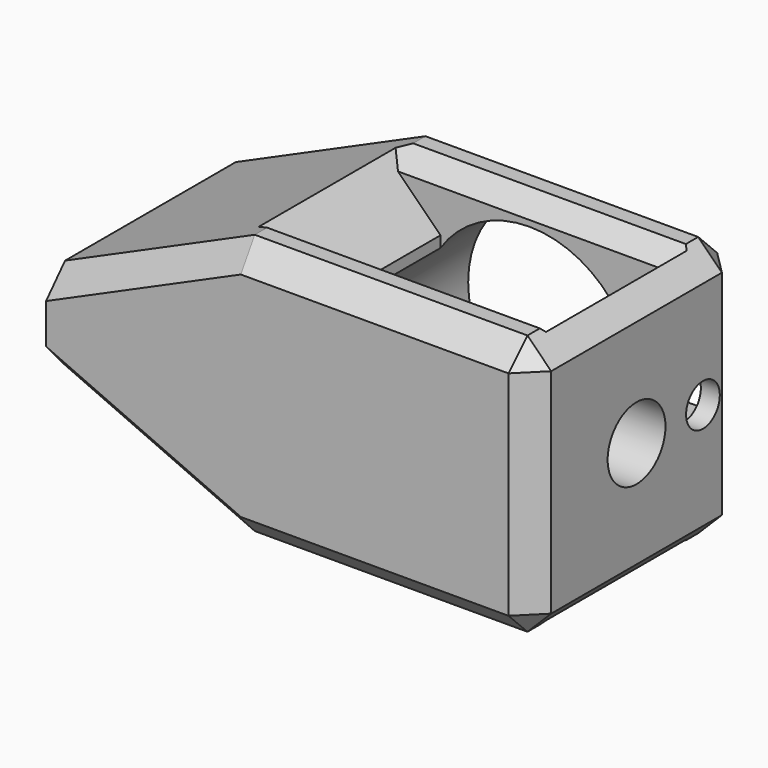
from build123d import *

# Parameters (mm, degrees)
F0_W          = 26
F0_H          = 22
F1_DEPTH      = 22
F2_R          = 9
F3_DEPTH      = 20
F4_W          = 15
F4_H          = 12.4
F5_DEPTH      = 22.001
F6_W          = 22
F6_H          = 22
F7_DEPTH      = 14
F8_W          = 18.7
F8_H          = 6
F9_DEPTH      = 12
F10_R         = 1.778
F11_DEPTH     = 40.001
F12_SIZE      = 1.5
F13_SIZE2     = 7.1236589649
F13_SIZE      = 16
F13_2_SIZE2   = 7.1236589649
F13_2_SIZE    = 16
F14_T1_DEPTH  = 27.800912408
F14_T3_DEPTH  = 27.800912408
F15_W         = 2.8
F15_H         = 5.8
F16_DEPTH     = 7
F17_W         = 22
F17_H         = 22
F18_DEPTH     = 1
F19_R         = 3.048
F20_DEPTH     = 26.5
F21_R         = 1.778
F22_DEPTH     = 6
F23_T1_DEPTH  = 2.5403411844
F23_T3_DEPTH  = 2.5403411844
F23_T5_DEPTH  = 2.5403411844
F23_T7_DEPTH  = 2.5403411844
F23_T9_DEPTH  = 32.2867319519
F23_T11_DEPTH = 32.2867319519
F23_T13_DEPTH = 30.3695452806
F24_T4_DEPTH  = 41.5282991577
F24_T10_DEPTH = 41.5282991577
F24_T16_DEPTH = 41.5282991577
F24_T22_DEPTH = 41.5282991577
F24_T28_DEPTH = 41.5282991577
F24_T34_DEPTH = 41.5282991577
F24_T40_DEPTH = 41.5282991577
F24_T46_DEPTH = 41.5282991577


# Not quite as in the source:
# - a fillet or chamfer that OpenCascade refuses, or shapes differently, is made with other operations: its cross-section is extruded or revolved along the edge and cut away or added


with BuildPart() as f1:
    # F0 (on Top) → F1 (new body)
    with BuildSketch(Plane.XY):
        with Locations((-0.9824799188, -2.7680952549)):
            Rectangle(F0_W, F0_H)
    extrude(amount=F1_DEPTH)

    # F2 (on face) → F3 (cut)
    with BuildSketch(Plane(origin=(0, 8.2319047451, 0), x_dir=(-1, 0, 0), z_dir=(0, 1, 0))):
        with Locations((0.9824799188, 11)):
            Circle(F2_R)
    extrude(amount=-F3_DEPTH, mode=Mode.SUBTRACT)

    # F4 (on face) → F5 (cut, through all)
    with BuildSketch(Plane.XY.offset(22)):
        with Locations((-0.9824799188, -2.7680952549)):
            Rectangle(F4_W, F4_H)
    extrude(amount=-F5_DEPTH, mode=Mode.SUBTRACT)

    # F6 (on face) → F7 (join)
    with BuildSketch(Plane(origin=(-13.9824799188, 0, 0), x_dir=(0, -1, 0), z_dir=(-1, 0, 0))):
        with Locations((2.7680952549, 11)):
            Rectangle(F6_W, F6_H)
    extrude(amount=F7_DEPTH)

    # F8 (on face) → F9 (cut)
    with BuildSketch(Plane(origin=(-27.9824799188, 0, 0), x_dir=(0, -1, 0), z_dir=(-1, 0, 0))):
        with Locations((2.7180952549, 11)):
            Rectangle(F8_W, F8_H)
    extrude(amount=-F9_DEPTH, mode=Mode.SUBTRACT)

    # F10 (on face) → F11 (cut, through all)
    with BuildSketch(Plane.YZ.offset(12.0175200812)):
        with Locations((-2.7180952549, 11)):
            Circle(F10_R)
    extrude(amount=-F11_DEPTH, mode=Mode.SUBTRACT)

    # F12
    f12_edges = [f1.edges().sort_by_distance(p)[0] for p in [
        (-0.98248, 3.431905, 22),
        (-0.98248, -8.968095, 22),
        (-0.98248, 3.431905, 0),
        (-0.98248, -8.968095, 0),
    ]]
    chamfer(f12_edges, length=F12_SIZE)

    # F13
    f13_edges = [f1.edges().sort_by_distance(p)[0] for p in [
        (-27.98248, -2.768095, 22),
    ]]
    f13_side = f1.faces().sort_by_distance((-10.474005, -2.768095, 22))[0]
    chamfer(f13_edges, length=F13_SIZE, length2=F13_SIZE2, reference=f13_side)

    # F13#2
    f13_2_edges = [f1.edges().sort_by_distance(p)[0] for p in [
        (-27.98248, -2.768095, 0),
    ]]
    f13_2_side = f1.faces().sort_by_distance((-10.474005, -2.768095, 0))[0]
    chamfer(f13_2_edges, length=F13_2_SIZE, length2=F13_2_SIZE2, reference=f13_2_side)

    # F14: chamfer of 2 on 4 edges, made by hand

    # F14_s2 → F14_t1 (cut)
    with BuildSketch(Plane(origin=(2.8731297183, 0, 1.2791997672), x_dir=(0, 1, 0), z_dir=(-0.9135454576, 0, -0.4067366431))):
        Polygon((8.2319047451, -22.971713726), (6.2319047451, -24.971713726), (8.2319047451, -24.971713726), align=None)
        Polygon((-11.7680952549, -24.971713726), (-13.7680952549, -22.971713726), (-13.7680952549, -24.971713726), align=None)
    extrude(amount=F14_T1_DEPTH, mode=Mode.SUBTRACT)

    # F14_s4 → F14_t3 (cut)
    with BuildSketch(Plane(origin=(-5.301463362, 0, 2.3603635629), x_dir=(0, 1, 0), z_dir=(-0.9135454576, 0, 0.4067366431))):
        Polygon((8.2319047451, 2.8737136579), (6.2319047451, 4.8737136579), (8.2319047451, 4.8737136579), align=None)
        Polygon((-11.7680952549, 4.8737136579), (-13.7680952549, 2.8737136579), (-13.7680952549, 4.8737136579), align=None)
    extrude(amount=F14_T3_DEPTH, mode=Mode.SUBTRACT)

    # F15 (on face) → F16 (cut)
    with BuildSketch(Plane(origin=(0, 8.2319047451, 0), x_dir=(-1, 0, 0), z_dir=(0, 1, 0))):
        with Locations((-10.0175200812, 11)):
            Rectangle(F15_W, F15_H)
    extrude(amount=-F16_DEPTH, mode=Mode.SUBTRACT)

    # F17 (on face) → F18 (join)
    with BuildSketch(Plane.YZ.offset(12.0175200812)):
        with Locations((-2.7680952549, 11)):
            Rectangle(F17_W, F17_H)
    extrude(amount=F18_DEPTH)

    # F19 (on face) → F20 (cut)
    with BuildSketch(Plane.YZ.offset(13.0175200812)):
        with Locations((-2.7680952549, 11)):
            Circle(F19_R)
    extrude(amount=-F20_DEPTH, mode=Mode.SUBTRACT)

    # F21 (on face) → F22 (cut)
    with BuildSketch(Plane.YZ.offset(13.0175200812)):
        with Locations((4.2319047451, 10.9924701974)):
            Circle(F21_R)
    extrude(amount=-F22_DEPTH, mode=Mode.SUBTRACT)

    # F23: chamfer of 2 on 8 edges, made by hand

    # F23_s2 → F23_t1 (cut)
    with BuildSketch(Plane(origin=(7.595205112, -7.595205112, -7.595205112), x_dir=(0.7071067812, 0.7071067812, 0), z_dir=(0.5773502692, -0.5773502692, -0.5773502692))):
        Polygon((-0.5307367951, 9.3021885081), (0.8834767672, 11.7516782509), (-1.9449503575, 11.7516782509), align=None)
    extrude(amount=F23_T1_DEPTH, mode=Mode.SUBTRACT)

    # F23_s4 → F23_t3 (cut)
    with BuildSketch(Plane(origin=(5.7498082754, 5.7498082754, -5.7498082754), x_dir=(-0.7071067812, 0.7071067812, 0), z_dir=(0.5773502692, 0.5773502692, -0.5773502692))):
        Polygon((-1.9697274939, 9.4915379396), (-3.3839410563, 7.0420481968), (-4.7981546187, 9.4915379396), align=None)
    extrude(amount=F23_T3_DEPTH, mode=Mode.SUBTRACT)

    # F23_s6 → F23_t5 (cut)
    with BuildSketch(Plane(origin=(13.0831416088, 13.0831416088, 13.0831416088), x_dir=(-0.7071067812, 0.7071067812, 0), z_dir=(0.5773502692, 0.5773502692, 0.5773502692))):
        Polygon((-1.9697274939, 8.4713868408), (-3.3839410563, 10.9208765836), (-4.7981546187, 8.4713868408), align=None)
    extrude(amount=F23_T5_DEPTH, mode=Mode.SUBTRACT)

    # F23_s8 → F23_t7 (cut)
    with BuildSketch(Plane(origin=(14.9285384454, -14.9285384454, 14.9285384454), x_dir=(0.7071067812, 0.7071067812, 0), z_dir=(0.5773502692, -0.5773502692, 0.5773502692))):
        Polygon((-0.5307367951, 8.6607362723), (0.8834767672, 6.2112465295), (-1.9449503575, 6.2112465295), align=None)
    extrude(amount=F23_T7_DEPTH, mode=Mode.SUBTRACT)

    # F23_s10 → F23_t9 (cut)
    with BuildSketch(Plane.XZ.offset(-13.375270721)):
        Polygon((11.0175200812, 0), (13.0175200812, 2), (13.0175200812, 0), align=None)
        Polygon((11.0175200812, 22), (13.0175200812, 20), (13.0175200812, 22), align=None)
    extrude(amount=F23_T9_DEPTH, mode=Mode.SUBTRACT)

    # F23_s12 → F23_t11 (cut)
    with BuildSketch(Plane.XY.offset(-5.1433659759)):
        Polygon((11.0175200812, 8.2319047451), (13.0175200812, 6.2319047451), (13.0175200812, 8.2319047451), align=None)
        Polygon((13.0175200812, -11.7680952549), (11.0175200812, -13.7680952549), (13.0175200812, -13.7680952549), align=None)
    extrude(amount=F23_T11_DEPTH, mode=Mode.SUBTRACT)

    # F23_s14 → F23_t13 (cut)
    with BuildSketch(Plane.YZ.offset(-12.2086592235)):
        Polygon((8.2319047451, 20), (6.2319047451, 22), (8.2319047451, 22), align=None)
        Polygon((-11.7680952549, 22), (-13.7680952549, 20), (-13.7680952549, 22), align=None)
        Polygon((-11.7680952549, 0), (-13.7680952549, 2), (-13.7680952549, 0), align=None)
        Polygon((8.2319047451, 2), (6.2319047451, 0), (8.2319047451, 0), align=None)
    extrude(amount=F23_T13_DEPTH, mode=Mode.SUBTRACT)

    # F24: chamfer of 5.08 on 4 edges, made by hand


with BuildPart() as f24_tool2:
    # F24_s3 → F24_t4 (new body)
    with BuildSketch(Plane.XZ.offset(23.5322448338)):
        Polygon((-8.4824799188, 16.92), (-13.5624799188, 22), (-8.4824799188, 22), align=None)
    extrude(amount=-F24_T4_DEPTH)

    split(bisect_by=Plane(origin=(0, 5.7659523726, 5.7659523726), x_dir=(1, 0, 0), z_dir=(0, 0.7071067812, 0.7071067812)), keep=Keep.TOP)

    split(bisect_by=Plane(origin=(0, -8.5340476274, 8.5340476274), x_dir=(1, 0, 0), z_dir=(0, -0.7071067812, 0.7071067812)), keep=Keep.TOP)


with BuildPart() as f1_1:
    add(f1.part)

    # F24_t1: cut F24_tool2
    add(f24_tool2.part, mode=Mode.SUBTRACT)


with BuildPart() as f24_tool8:
    # F24_s9 → F24_t10 (new body)
    with BuildSketch(Plane.XZ.offset(23.5322448338)):
        Polygon((-8.4824799188, 16.92), (-13.5624799188, 22), (-8.4824799188, 22), align=None)
    extrude(amount=-F24_T10_DEPTH)

    split(bisect_by=Plane.XZ.offset(8.9680952549), keep=Keep.BOTTOM)

    split(bisect_by=Plane.XZ.offset(-3.4319047451), keep=Keep.TOP)


with BuildPart() as f1_2:
    add(f1_1.part)

    # F24_t7: cut F24_tool8
    add(f24_tool8.part, mode=Mode.SUBTRACT)


with BuildPart() as f24_tool14:
    # F24_s15 → F24_t16 (new body)
    with BuildSketch(Plane.XZ.offset(-17.996054324)):
        Polygon((6.5175200812, 16.92), (11.5975200812, 22), (6.5175200812, 22), align=None)
    extrude(amount=F24_T16_DEPTH)

    split(bisect_by=Plane(origin=(0, 5.7659523726, 5.7659523726), x_dir=(1, 0, 0), z_dir=(0, 0.7071067812, 0.7071067812)), keep=Keep.TOP)

    split(bisect_by=Plane(origin=(0, -8.5340476274, 8.5340476274), x_dir=(1, 0, 0), z_dir=(0, -0.7071067812, 0.7071067812)), keep=Keep.TOP)


with BuildPart() as f1_3:
    add(f1_2.part)

    # F24_t13: cut F24_tool14
    add(f24_tool14.part, mode=Mode.SUBTRACT)


with BuildPart() as f24_tool20:
    # F24_s21 → F24_t22 (new body)
    with BuildSketch(Plane.XZ.offset(-17.996054324)):
        Polygon((6.5175200812, 16.92), (11.5975200812, 22), (6.5175200812, 22), align=None)
    extrude(amount=F24_T22_DEPTH)

    split(bisect_by=Plane.XZ.offset(8.9680952549), keep=Keep.BOTTOM)

    split(bisect_by=Plane.XZ.offset(-3.4319047451), keep=Keep.TOP)


with BuildPart() as f1_4:
    add(f1_3.part)

    # F24_t19: cut F24_tool20
    add(f24_tool20.part, mode=Mode.SUBTRACT)


with BuildPart() as f24_tool26:
    # F24_s27 → F24_t28 (new body)
    with BuildSketch(Plane.XZ.offset(23.5322448338)):
        Polygon((11.5975200812, 0), (6.5175200812, 5.08), (6.5175200812, 0), align=None)
    extrude(amount=-F24_T28_DEPTH)

    split(bisect_by=Plane.XZ.offset(8.9680952549), keep=Keep.BOTTOM)

    split(bisect_by=Plane(origin=(0, 2.4659523726, 2.4659523726), x_dir=(1, 0, 0), z_dir=(0, -0.7071067812, -0.7071067812)), keep=Keep.TOP)


with BuildPart() as f1_5:
    add(f1_4.part)

    # F24_t25: cut F24_tool26
    add(f24_tool26.part, mode=Mode.SUBTRACT)


with BuildPart() as f24_tool32:
    # F24_s33 → F24_t34 (new body)
    with BuildSketch(Plane.XZ.offset(23.5322448338)):
        Polygon((11.5975200812, 0), (6.5175200812, 5.08), (6.5175200812, 0), align=None)
    extrude(amount=-F24_T34_DEPTH)

    split(bisect_by=Plane.XZ.offset(-3.4319047451), keep=Keep.TOP)

    split(bisect_by=Plane(origin=(0, -5.2340476274, 5.2340476274), x_dir=(1, 0, 0), z_dir=(0, 0.7071067812, -0.7071067812)), keep=Keep.TOP)


with BuildPart() as f1_6:
    add(f1_5.part)

    # F24_t31: cut F24_tool32
    add(f24_tool32.part, mode=Mode.SUBTRACT)


with BuildPart() as f24_tool38:
    # F24_s39 → F24_t40 (new body)
    with BuildSketch(Plane.XZ.offset(-17.996054324)):
        Polygon((-13.5624799188, 0), (-8.4824799188, 5.08), (-8.4824799188, 0), align=None)
    extrude(amount=F24_T40_DEPTH)

    split(bisect_by=Plane.XZ.offset(-3.4319047451), keep=Keep.TOP)

    split(bisect_by=Plane(origin=(0, -5.2340476274, 5.2340476274), x_dir=(1, 0, 0), z_dir=(0, 0.7071067812, -0.7071067812)), keep=Keep.TOP)


with BuildPart() as f1_7:
    add(f1_6.part)

    # F24_t37: cut F24_tool38
    add(f24_tool38.part, mode=Mode.SUBTRACT)


with BuildPart() as f24_tool44:
    # F24_s45 → F24_t46 (new body)
    with BuildSketch(Plane.XZ.offset(-17.996054324)):
        Polygon((-13.5624799188, 0), (-8.4824799188, 5.08), (-8.4824799188, 0), align=None)
    extrude(amount=F24_T46_DEPTH)

    split(bisect_by=Plane.XZ.offset(8.9680952549), keep=Keep.BOTTOM)

    split(bisect_by=Plane(origin=(0, 2.4659523726, 2.4659523726), x_dir=(1, 0, 0), z_dir=(0, -0.7071067812, -0.7071067812)), keep=Keep.TOP)


with BuildPart() as f1_8:
    add(f1_7.part)

    # F24_t43: cut F24_tool44
    add(f24_tool44.part, mode=Mode.SUBTRACT)


solid = f1_8.part
